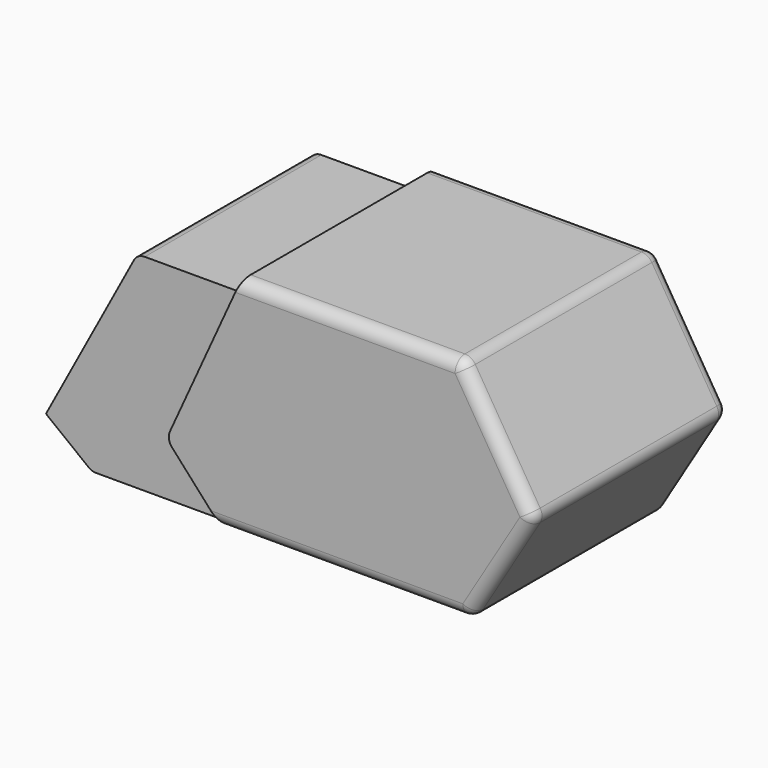
from build123d import *

# Parameters (mm, degrees)
F1_DEPTH      = 50
F1_DEPTH_BACK = 50
F2_DEPTH      = 45
F2_DEPTH_BACK = 45
F3_T          = -2.5
F4_T1_DEPTH   = 99.870741826
F4_T3_DEPTH   = 110.7687976219
F4_T5_DEPTH   = 90
F4_T7_DEPTH   = 50.4710288906
F4_T9_DEPTH   = 45.1571225653
F4_T11_DEPTH  = 13.1936213228
F4_T13_DEPTH  = 13.1936213228
F4_T15_DEPTH  = 94.7250280473
F4_T17_DEPTH  = 104.9542642721
F4_T19_DEPTH  = 98.5632481835
F4_T24_DEPTH  = 5.1
F4_T30_DEPTH  = 5.1
F4_T36_DEPTH  = 5.1
F4_T42_DEPTH  = 5.1
F4_T48_DEPTH  = 5.1
F4_T54_DEPTH  = 5.1


# Not quite as in the source:
# - a fillet or chamfer that OpenCascade refuses, or shapes differently, is made with other operations: its cross-section is extruded or revolved along the edge and cut away or added


with BuildPart() as f1:
    # F0 (on Front) → F1 (new body, two sides)
    with BuildSketch(Plane.XZ) as f1_sk:
        Polygon((-26.3700434903, -45.8344183862), (74.724436402, -45.8344183862), (101.0472456507, -2.1214453581), (71.5359502951, 45.8344183862), (-18.6287677695, 45.8344183862), (-22.0811308447, 38.2426545129), (-48.933561855, -20.8059771664), align=None)
    extrude(amount=F1_DEPTH)
    extrude(f1_sk.sketch, amount=-F1_DEPTH_BACK)

    # F0 (on Front) → F2 (join, two sides)
    with BuildSketch(Plane.XZ) as f2_sk:
        Polygon((-83.371719636, -45.8344183862), (-26.3700434903, -45.8344183862), (-48.933561855, -20.8059771664), (-22.0811308447, 38.2426545129), (-64.8318102514, 38.2426545129), (-102.0922288299, -31.1698793042), (-102.0922288299, -31.3050675487), align=None)
    extrude(amount=F2_DEPTH)
    extrude(f2_sk.sketch, amount=-F2_DEPTH_BACK)

    # F3
    f3_openings = [f1.faces().sort_by_distance(p)[0] for p in [
        (-83.46202, 0, 3.536388),
    ]]
    offset(amount=F3_T, openings=f3_openings, kind=Kind.INTERSECTION)

    # F4: fillet of radius 5 on 16 edges, made by hand

    # F4_s2 → F4_t1 (cut)
    with BuildSketch(Plane.YZ.offset(-31.1287677695)):
        with BuildLine():
            ThreePointArc((-50, 40.8344183862), (-48.5355339059, 44.3699522922), (-45, 45.8344183862))
            Line((-45, 45.8344183862), (-50, 45.8344183862))
            Line((-50, 45.8344183862), (-50, 40.8344183862))
        make_face()
        with BuildLine():
            ThreePointArc((45, 45.8344183862), (48.5355339059, 44.3699522922), (50, 40.8344183862))
            Line((50, 40.8344183862), (50, 45.8344183862))
            Line((50, 45.8344183862), (45, 45.8344183862))
        make_face()
    extrude(amount=F4_T1_DEPTH, mode=Mode.SUBTRACT)

    # F4_s4 → F4_t3 (cut)
    with BuildSketch(Plane.YZ.offset(-38.8700434903)):
        with BuildLine():
            ThreePointArc((-50, -40.8344183862), (-48.5355339059, -44.3699522922), (-45, -45.8344183862))
            Line((-45, -45.8344183862), (-50, -45.8344183862))
            Line((-50, -45.8344183862), (-50, -40.8344183862))
        make_face()
        with BuildLine():
            ThreePointArc((50, -40.8344183862), (48.5355339059, -44.3699522922), (45, -45.8344183862))
            Line((45, -45.8344183862), (50, -45.8344183862))
            Line((50, -45.8344183862), (50, -40.8344183862))
        make_face()
    extrude(amount=F4_T3_DEPTH, mode=Mode.SUBTRACT)

    # F4_s6 → F4_t5 (cut)
    with BuildSketch(Plane.XZ.offset(-45)):
        with BuildLine():
            ThreePointArc((73.0002658545, 43.4549051661), (71.1809867769, 45.1991883629), (68.7419740565, 45.8344183862))
            Line((68.7419740565, 45.8344183862), (71.5359502951, 45.8344183862))
            Line((71.5359502951, 45.8344183862), (73.0002658545, 43.4549051661))
        make_face()
        with BuildLine():
            ThreePointArc((99.4519986494, 0.4708314943), (100.1936487884, -2.1255590928), (99.4770580597, -4.7289773721))
            Line((99.4770580597, -4.7289773721), (101.0472456507, -2.1214453581))
            Line((101.0472456507, -2.1214453581), (99.4519986494, 0.4708314943))
        make_face()
        with BuildLine():
            ThreePointArc((76.1821053399, -43.4137404728), (74.3587733965, -45.1873834925), (71.8987541316, -45.8344183862))
            Line((71.8987541316, -45.8344183862), (74.724436402, -45.8344183862))
            Line((74.724436402, -45.8344183862), (76.1821053399, -43.4137404728))
        make_face()
    extrude(amount=F4_T5_DEPTH, mode=Mode.SUBTRACT)

    # F4_s8 → F4_t7 (cut)
    with BuildSketch(Plane(origin=(27.1071233885, 0, -44.0490835816), x_dir=(0, 1, 0), z_dir=(-0.524097356, 0, 0.8516583596))):
        with BuildLine():
            ThreePointArc((-45, -84.945887569), (-48.5355339059, -83.4814214749), (-50, -79.945887569))
            Line((-50, -79.945887569), (-50, -84.945887569))
            Line((-50, -84.945887569), (-45, -84.945887569))
        make_face()
        with BuildLine():
            ThreePointArc((45, -84.945887569), (48.5355339059, -83.4814214749), (50, -79.945887569))
            Line((50, -79.945887569), (50, -84.945887569))
            Line((50, -84.945887569), (45, -84.945887569))
        make_face()
    extrude(amount=F4_T7_DEPTH, mode=Mode.SUBTRACT)

    # F4_s10 → F4_t9 (cut)
    with BuildSketch(Plane(origin=(1.0876371054, 0, 1.8061845528), x_dir=(0, 1, 0), z_dir=(0.5158644173, 0, 0.8566702417))):
        with BuildLine():
            ThreePointArc((-45, -87.6585465243), (-48.5355339059, -86.1940804302), (-50, -82.6585465243))
            Line((-50, -82.6585465243), (-50, -87.6585465243))
            Line((-50, -87.6585465243), (-45, -87.6585465243))
        make_face()
        with BuildLine():
            ThreePointArc((45, -87.6585465243), (48.5355339059, -86.1940804302), (50, -82.6585465243))
            Line((50, -82.6585465243), (50, -87.6585465243))
            Line((50, -87.6585465243), (45, -87.6585465243))
        make_face()
    extrude(amount=F4_T9_DEPTH, mode=Mode.SUBTRACT)

    # F4_s12 → F4_t11 (cut)
    with BuildSketch(Plane.XZ.offset(-58.1936213228)):
        with BuildLine():
            ThreePointArc((-47.5768355145, -17.8225290777), (-47.9666216966, -20.6564474707), (-46.7390274483, -23.2402506923))
            Line((-46.7390274483, -23.2402506923), (-48.933561855, -20.8059771664))
            Line((-48.933561855, -20.8059771664), (-47.5768355145, -17.8225290777))
        make_face()
    extrude(amount=F4_T11_DEPTH, mode=Mode.SUBTRACT)

    # F4_s14 → F4_t13 (cut)
    with BuildSketch(Plane.XZ.offset(45)):
        with BuildLine():
            ThreePointArc((-47.5768355145, -17.8225290777), (-47.9666216966, -20.6564474707), (-46.7390274483, -23.2402506923))
            Line((-46.7390274483, -23.2402506923), (-48.933561855, -20.8059771664))
            Line((-48.933561855, -20.8059771664), (-47.5768355145, -17.8225290777))
        make_face()
    extrude(amount=F4_T13_DEPTH, mode=Mode.SUBTRACT)

    # F4_s16 → F4_t15 (cut)
    with BuildSketch(Plane.XZ.offset(-47.3625140236)):
        with BuildLine():
            ThreePointArc((-101.3456869873, -31.8844731745), (-101.7374694613, -31.5465154042), (-102.0922288299, -31.1698793042))
            Line((-102.0922288299, -31.1698793042), (-102.0922288299, -31.3050675487))
            Line((-102.0922288299, -31.3050675487), (-101.3456869873, -31.8844731745))
        make_face()
    extrude(amount=F4_T15_DEPTH, mode=Mode.SUBTRACT)

    # F4_s18 → F4_t17 (cut)
    with BuildSketch(Plane.XZ.offset(-52.477132136)):
        with BuildLine():
            ThreePointArc((-61.840957397, 38.2426545129), (-64.4076618274, 37.5335784655), (-66.2463708048, 35.6074658598))
            Line((-66.2463708048, 35.6074658598), (-64.8318102514, 38.2426545129))
            Line((-64.8318102514, 38.2426545129), (-61.840957397, 38.2426545129))
        make_face()
    extrude(amount=F4_T17_DEPTH, mode=Mode.SUBTRACT)

    # F4_s20 → F4_t19 (cut)
    with BuildSketch(Plane.XZ.offset(-49.2816240917)):
        with BuildLine():
            ThreePointArc((-81.6590699993, -45.8344183862), (-83.2793065621, -45.5646227667), (-84.7246900339, -44.7843517785))
            Line((-84.7246900339, -44.7843517785), (-83.371719636, -45.8344183862))
            Line((-83.371719636, -45.8344183862), (-81.6590699993, -45.8344183862))
        make_face()
    extrude(amount=F4_T19_DEPTH, mode=Mode.SUBTRACT)


with BuildPart() as f4_tool22:
    # F4_s23 → F4_t24 (new body)
    with BuildSketch(Plane.XZ.offset(45)):
        Polygon((68.7419740565, 40.8344183862), (68.7419740565, 45.9344183862), (71.5918298199, 45.9344183862), (73.0854316904, 43.5073149017), align=None)
    extrude(amount=F4_T24_DEPTH)

    # F4_s25 → F4_t26 (revolve, cut)
    with BuildSketch(Plane(origin=(68.7419740565, -45, 40.8344183862), x_dir=(-0.4878025441, 0, -0.8729539953), z_dir=(-0.8729539953, 0, 0.4878025441))):
        with BuildLine():
            ThreePointArc((0, -5), (5, 0), (0, 5))
            Line((0, 5), (0, -5))
        make_face()
    revolve(axis=Axis((68.7419740565, -45, 40.8344183862), (0, -1, 0)), mode=Mode.SUBTRACT)


with BuildPart() as f1_1:
    add(f1.part)

    # F4_t21: cut F4_tool22
    add(f4_tool22.part, mode=Mode.SUBTRACT)


with BuildPart() as f4_tool28:
    # F4_s29 → F4_t30 (new body)
    with BuildSketch(Plane.XZ.offset(45)):
        Polygon((71.8987541316, -40.8344183862), (71.8987541316, -45.9344183862), (74.7809500474, -45.9344183862), (76.2677723641, -43.4653269145), align=None)
    extrude(amount=F4_T30_DEPTH)

    # F4_s31 → F4_t32 (revolve, cut)
    with BuildSketch(Plane(origin=(71.8987541316, -45, -40.8344183862), x_dir=(-0.492003853, 0, 0.8705930213), z_dir=(0.8705930213, 0, 0.492003853))):
        with BuildLine():
            ThreePointArc((0, -5), (5, 0), (0, 5))
            Line((0, 5), (0, -5))
        make_face()
    revolve(axis=Axis((71.8987541316, -45, -40.8344183862), (0, -1, 0)), mode=Mode.SUBTRACT)


with BuildPart() as f1_2:
    add(f1_1.part)

    # F4_t27: cut F4_tool28
    add(f4_tool28.part, mode=Mode.SUBTRACT)


with BuildPart() as f4_tool34:
    # F4_s35 → F4_t36 (new body)
    with BuildSketch(Plane.XZ.offset(-45)):
        Polygon((68.7419740565, 40.8344183862), (73.0854316904, 43.5073149017), (71.5918298199, 45.9344183862), (68.7419740565, 45.9344183862), align=None)
    extrude(amount=-F4_T36_DEPTH)

    # F4_s37 → F4_t38 (revolve, cut)
    with BuildSketch(Plane(origin=(68.7419740565, 45, 40.8344183862), x_dir=(-0.4878025441, 0, -0.8729539953), z_dir=(0.8729539953, 0, -0.4878025441))):
        with BuildLine():
            ThreePointArc((0, -5), (5, 0), (0, 5))
            Line((0, 5), (0, -5))
        make_face()
    revolve(axis=Axis((68.7419740565, 45, 40.8344183862), (0, 1, 0)), mode=Mode.SUBTRACT)


with BuildPart() as f1_3:
    add(f1_2.part)

    # F4_t33: cut F4_tool34
    add(f4_tool34.part, mode=Mode.SUBTRACT)


with BuildPart() as f4_tool40:
    # F4_s41 → F4_t42 (new body)
    with BuildSketch(Plane.XZ.offset(-45)):
        Polygon((71.8987541316, -40.8344183862), (71.8987541316, -45.9344183862), (74.7809500474, -45.9344183862), (76.2677723641, -43.4653269145), align=None)
    extrude(amount=-F4_T42_DEPTH)

    # F4_s43 → F4_t44 (revolve, cut)
    with BuildSketch(Plane(origin=(71.8987541316, 45, -40.8344183862), x_dir=(-0.492003853, 0, 0.8705930213), z_dir=(-0.8705930213, 0, -0.492003853))):
        with BuildLine():
            ThreePointArc((0, -5), (5, 0), (0, 5))
            Line((0, 5), (0, -5))
        make_face()
    revolve(axis=Axis((71.8987541316, 45, -40.8344183862), (0, 1, 0)), mode=Mode.SUBTRACT)


with BuildPart() as f1_4:
    add(f1_3.part)

    # F4_t39: cut F4_tool40
    add(f4_tool40.part, mode=Mode.SUBTRACT)


with BuildPart() as f4_tool46:
    # F4_s47 → F4_t48 (new body)
    with BuildSketch(Plane.XZ.offset(45)):
        Polygon((95.1937068514, -2.1496552855), (99.5371644853, 0.5232412299), (101.1643164267, -2.1208811596), (99.5627250839, -4.7805638139), align=None)
    extrude(amount=F4_T48_DEPTH)

    # F4_s49 → F4_t50 (revolve, cut)
    with BuildSketch(Plane(origin=(95.1937068514, -45, -2.1496552855), x_dir=(-0.9999883874, 0, -0.0048192386), z_dir=(-0.0048192386, 0, 0.9999883874))):
        with BuildLine():
            ThreePointArc((0, -5), (5, 0), (0, 5))
            Line((0, 5), (0, -5))
        make_face()
    revolve(axis=Axis((95.1937068514, -45, -2.1496552855), (0, -1, 0)), mode=Mode.SUBTRACT)


with BuildPart() as f1_5:
    add(f1_4.part)

    # F4_t45: cut F4_tool46
    add(f4_tool46.part, mode=Mode.SUBTRACT)


with BuildPart() as f4_tool52:
    # F4_s53 → F4_t54 (new body)
    with BuildSketch(Plane.XZ.offset(-45)):
        Polygon((95.1937068514, -2.1496552855), (99.5371644853, 0.5232412299), (101.1643164267, -2.1208811596), (99.5627250839, -4.7805638139), align=None)
    extrude(amount=-F4_T54_DEPTH)

    # F4_s55 → F4_t56 (revolve, cut)
    with BuildSketch(Plane(origin=(95.1937068514, 45, -2.1496552855), x_dir=(-0.9999883874, 0, -0.0048192386), z_dir=(0.0048192386, 0, -0.9999883874))):
        with BuildLine():
            ThreePointArc((0, -5), (5, 0), (0, 5))
            Line((0, 5), (0, -5))
        make_face()
    revolve(axis=Axis((95.1937068514, 45, -2.1496552855), (0, 1, 0)), mode=Mode.SUBTRACT)


with BuildPart() as f1_6:
    add(f1_5.part)

    # F4_t51: cut F4_tool52
    add(f4_tool52.part, mode=Mode.SUBTRACT)


solid = f1_6.part
